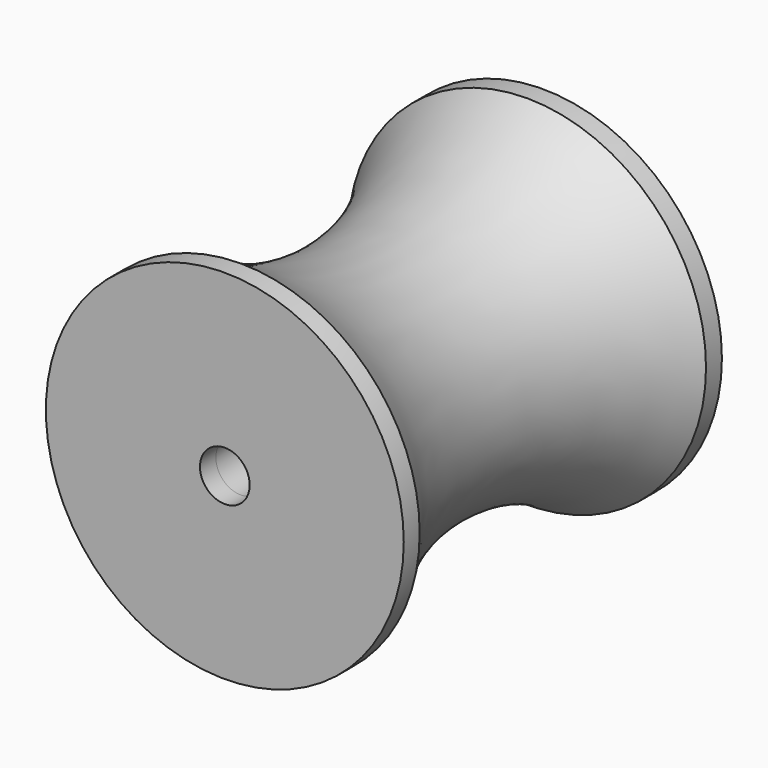
from build123d import *

# Parameters (mm, degrees)
F2_R     = 11.43
F2_R_2   = 1.5875
F3_DEPTH = 1.27
F5_R     = 11.43
F5_R_2   = 1.5875
F6_DEPTH = 1.27


# Not quite as in the source:
# - a variable given as a bare number and used for a length is read in inches; the dataset says mm whatever the document's units were


with BuildPart() as f3:
    # F2 (on offset) → F3 (new body)
    with BuildSketch(Plane.XZ.offset(11.43)):
        Circle(F2_R)
        Circle(F2_R_2, mode=Mode.SUBTRACT)
    extrude(amount=F3_DEPTH)



with BuildPart() as f6:
    # F5 (on offset) → F6 (new body)
    with BuildSketch(Plane.XZ.offset(-11.43)):
        Circle(F5_R)
        Circle(F5_R_2, mode=Mode.SUBTRACT)
    extrude(amount=-F6_DEPTH)


with BuildPart() as f3_1:
    add(f3.part)

    add(f6.part)  # F8 merges F6
    # F7 (on Right) → F8 (revolve)
    with BuildSketch(Plane.YZ):
        with BuildLine():
            ThreePointArc((11.43, 11.43), (0, 7.8646021863), (-11.43, 11.43))
            Line((-11.43, 11.43), (-11.43, 1.5875))
            Line((-11.43, 1.5875), (11.43, 1.5875))
            Line((11.43, 1.5875), (11.43, 11.43))
        make_face()
    revolve(axis=Axis((0, 0, 0), (0, -1, 0)))


solid = f3_1.part
